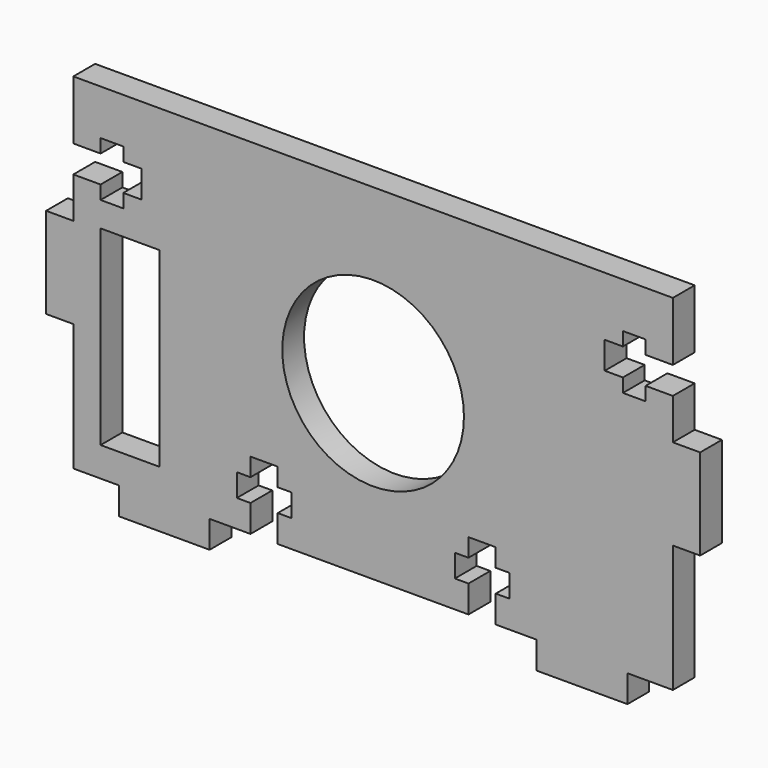
from build123d import *

# Parameters (mm, degrees)
F0_W     = 6.5
F0_H     = 21
F0_R     = 10
F1_DEPTH = 3
F3_DEPTH = 3


# Not quite as in the source:
# - a feature names something its author has since deleted; it is built from what else it names


with BuildPart() as f1:
    # F0 (on Front) → F1 (new body)
    with BuildSketch(Plane.XZ):
        Polygon((33, 5), (33, 19), (-33, 19), (-33, 5), (-36, 5), (-36, -5), (-33, -5), (-33, -19), (-28, -19), (-28, -22), (-18, -22), (-18, -19), (0, -19), (18, -19), (18, -22), (28, -22), (28, -19), (33, -19), (33, -5), (36, -5), (36, 5), align=None)
        with Locations((-26.75, -5.25)):
            Rectangle(F0_W, F0_H, mode=Mode.SUBTRACT)
        Circle(F0_R, mode=Mode.SUBTRACT)
    extrude(amount=F1_DEPTH)

    # F2 (on face) → F3 (cut, through all)
    with BuildSketch(Plane.XZ.offset(3)):
        Polygon((10.5, -16), (10.5, -19), (13.5, -19), (13.5, -16), (15, -16), (15, -13.5), (13.5, -13.5), (13.5, -11.5), (10.5, -11.5), (10.5, -13.5), (9, -13.5), (9, -16), align=None)
        Polygon((30, 9.5), (33, 9.5), (33, 12.5), (30, 12.5), (30, 14), (27.5, 14), (27.5, 12.5), (25.5, 12.5), (25.5, 9.5), (27.5, 9.5), (27.5, 8), (30, 8), align=None)
        Polygon((-33, 12.5), (-33, 9.5), (-30, 9.5), (-30, 8), (-27.5, 8), (-27.5, 9.5), (-25.5, 9.5), (-25.5, 12.5), (-27.5, 12.5), (-27.5, 14), (-30, 14), (-30, 12.5), align=None)
        Polygon((-13.5, -19), (-10.5, -19), (-10.5, -16), (-9, -16), (-9, -13.5), (-10.5, -13.5), (-10.5, -11.5), (-13.5, -11.5), (-13.5, -13.5), (-15, -13.5), (-15, -16), (-13.5, -16), align=None)
    extrude(amount=-F3_DEPTH, mode=Mode.SUBTRACT)


solid = f1.part
